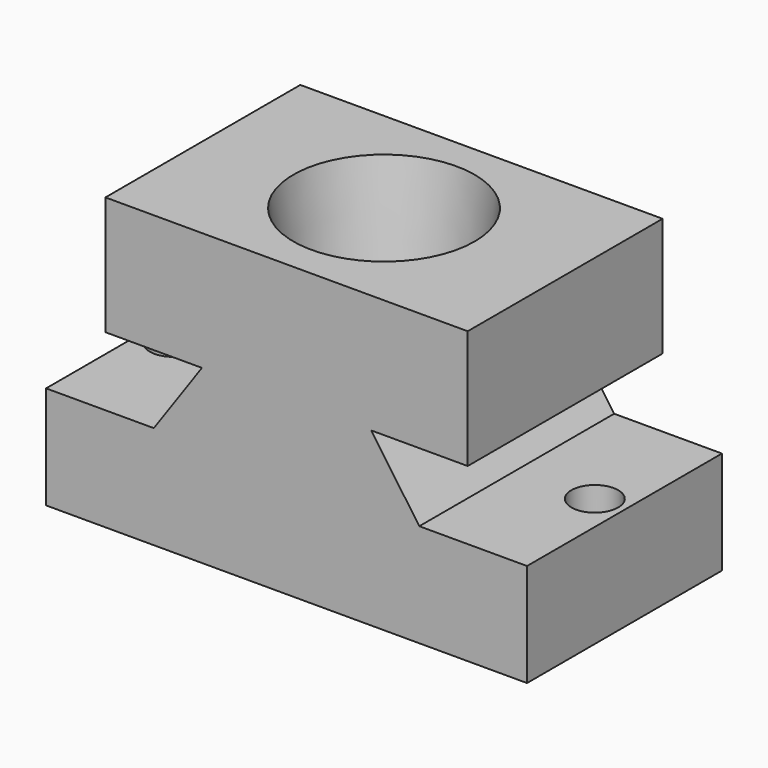
from build123d import *

# Parameters (mm, degrees)
F0_W      = 154
F0_H      = 78
F1_DEPTH  = 46.5
F3_DEPTH  = 80
F4_R      = 7.5
F5_DEPTH  = 50
F6_R      = 29
F7_DEPTH  = 30
F8_SIZE2  = 3.99999
F8_SIZE   = 29.99999
F9_R      = 7.5
F10_DEPTH = 40


# Not quite as in the source:
# - a fillet or chamfer is up to 0.001 mm smaller than in the source, because OpenCascade refuses the exact size


with BuildPart() as f1:
    # F0 (on Top) → F1 (new body, symmetric)
    with BuildSketch(Plane.XY):
        Rectangle(F0_W, F0_H)
    extrude(amount=F1_DEPTH, both=True)

    # F2 (on face) → F3 (cut)
    with BuildSketch(Plane.XZ.offset(39)):
        Polygon((-77, 46.5), (-77, -13.5), (-42.5, -13.5), (-27.0954341594, 8.5), (-58, 8.5), (-58, 46.5), align=None)
        Polygon((77, 46.5), (58, 46.5), (58, 8.5), (27.0954341594, 8.5), (42.5, -13.5), (77, -13.5), align=None)
    extrude(amount=-F3_DEPTH, mode=Mode.SUBTRACT)

    # F4 (on face) → F5 (cut)
    with BuildSketch(Plane.XY.offset(-13.5)):
        with Locations((-67.5, 0)):
            Circle(F4_R)
    extrude(amount=-F5_DEPTH, mode=Mode.SUBTRACT)

    # F6 (on face) → F7 (cut)
    with BuildSketch(Plane.XY.offset(46.5)):
        Circle(F6_R)
    extrude(amount=-F7_DEPTH, mode=Mode.SUBTRACT)

    # F8 (size 30 and 4 in the source; OpenCascade refuses exactly that, so slightly less here)
    f8_edges = [f1.edges().sort_by_distance(p)[0] for p in [
        (-29, 0, 16.5),
    ]]
    f8_side = f1.faces().sort_by_distance((-29, 0, 31.5))[0]
    chamfer(f8_edges, length=F8_SIZE, length2=F8_SIZE2, reference=f8_side)

    # F9 (on face) → F10 (cut)
    with BuildSketch(Plane.XY.offset(-13.5)):
        with Locations((67.5, 0)):
            Circle(F9_R)
    extrude(amount=-F10_DEPTH, mode=Mode.SUBTRACT)


solid = f1.part
